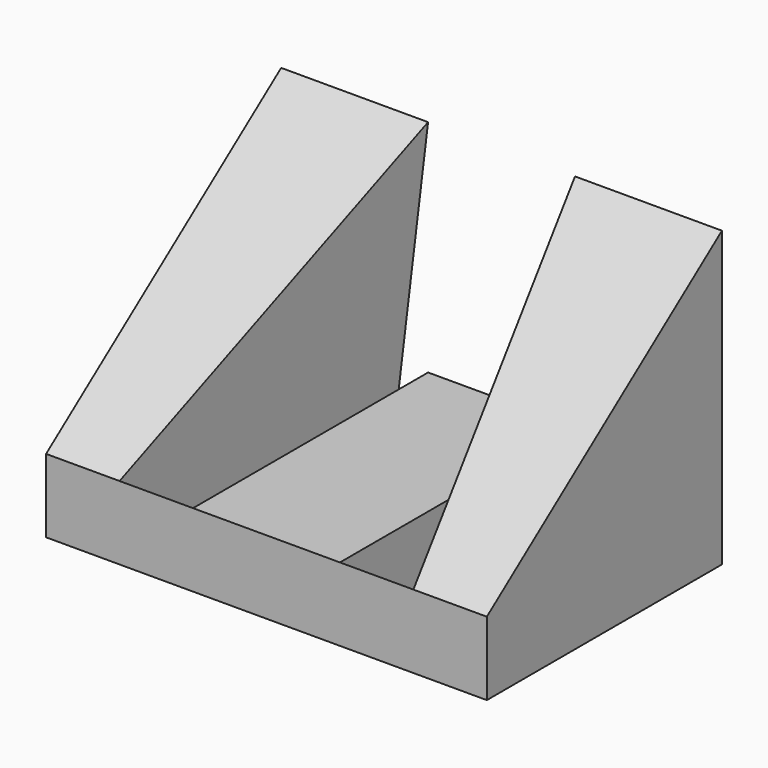
from build123d import *

# Parameters (mm, degrees)
F0_W     = 60
F0_H     = 40
F1_DEPTH = 40
F2_W     = 20
F2_H     = 30
F3_DEPTH = 40
F5_DEPTH = 60
F8_DEPTH = 40


# Not quite as in the source:
# - a feature of the source that left no trace in its solid (it failed there, or was rolled back) is left out


with BuildPart() as f1:
    # F0 (on Front) → F1 (new body)
    with BuildSketch(Plane.XZ):
        with Locations((30, 20)):
            Rectangle(F0_W, F0_H)
    extrude(amount=F1_DEPTH)

    # F2 (on face) → F3 (cut)
    with BuildSketch(Plane.XZ.offset(40)):
        with Locations((30, 25)):
            Rectangle(F2_W, F2_H)
    extrude(amount=-F3_DEPTH, mode=Mode.SUBTRACT)

    # F4 (on face) → F5 (cut)
    with BuildSketch(Plane.YZ.offset(60)):
        Polygon((-40, 40), (-40, 10), (0, 40), align=None)
    extrude(amount=-F5_DEPTH, mode=Mode.SUBTRACT)

    # F6 (on face) + F7 (on face) → F8 (cut)
    with BuildSketch(Plane(origin=(0, -19.2, 25.6), x_dir=(1, 0, 0), z_dir=(0, -0.6, 0.8))):
        Polygon((20, -26), (20, 24), (10, -26), align=None)
    with BuildSketch(Plane(origin=(0, -19.2, 25.6), x_dir=(1, 0, 0), z_dir=(0, -0.6, 0.8))):
        Polygon((50, -26), (40, 24), (40, -26), align=None)
    extrude(amount=-F8_DEPTH, mode=Mode.SUBTRACT)


solid = f1.part
